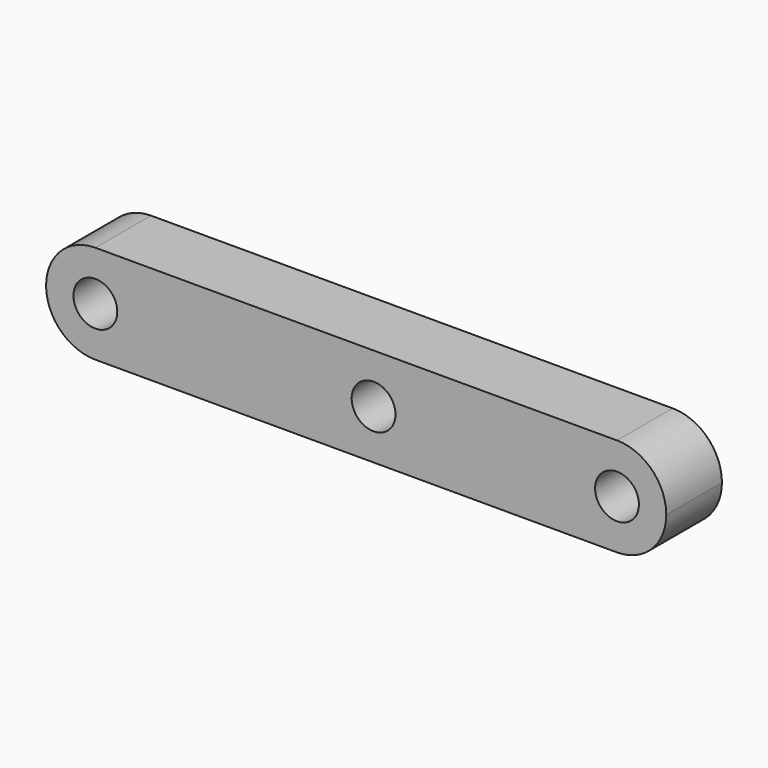
from build123d import *

# Parameters (mm, degrees)
F0_R     = 4
F1_DEPTH = 12.7


# Not quite as in the source:
# - a feature names something its author has since deleted; it is built from what else it names


with BuildPart() as f1:
    # F0 (on Front) → F1 (new body)
    with BuildSketch(Plane.XZ):
        with BuildLine():
            ThreePointArc((-50.8, -9), (-44.4360389693, -6.3639610307), (-41.8, 0))
            ThreePointArc((-41.8, 0), (-44.4360389693, 6.3639610307), (-50.8, 9))
            ThreePointArc((-50.8, 9), (-59.8, 0), (-50.8, -9))
        make_face()
        with Locations((-50.8, 0)):
            Circle(F0_R, mode=Mode.SUBTRACT)
        with BuildLine():
            ThreePointArc((9, 0), (6.3639610238, 6.3639610375), (-1.93e-08, 9))
            ThreePointArc((-1.93e-08, 9), (-9, -9.7e-09), (0, -9))
            ThreePointArc((0, -9), (6.3639610307, -6.3639610307), (9, 0))
        make_face()
        Circle(F0_R, mode=Mode.SUBTRACT)
        with BuildLine():
            ThreePointArc((-50.8, 9), (-44.4360389693, 6.3639610307), (-41.8, 0))
            ThreePointArc((-41.8, 0), (-44.4360389693, -6.3639610307), (-50.8, -9))
            Line((-50.8, -9), (0, -9))
            ThreePointArc((0, -9), (-9, -9.7e-09), (-1.93e-08, 9))
            Line((-1.93e-08, 9), (-50.8, 9))
        make_face()
        with BuildLine():
            Line((44.45, 9), (-1.93e-08, 9))
            ThreePointArc((-1.93e-08, 9), (6.3639610238, 6.3639610375), (9, 0))
            ThreePointArc((9, 0), (6.3639610307, -6.3639610307), (0, -9))
            Line((0, -9), (44.45, -9))
            ThreePointArc((44.45, -9), (35.45, 0), (44.45, 9))
        make_face()
        with BuildLine():
            ThreePointArc((53.45, 0), (50.8139610307, 6.3639610307), (44.45, 9))
            ThreePointArc((44.45, 9), (35.45, 0), (44.45, -9))
            ThreePointArc((44.45, -9), (50.8139610307, -6.3639610307), (53.45, 0))
        make_face()
        with Locations((44.45, 0)):
            Circle(F0_R, mode=Mode.SUBTRACT)
    extrude(amount=F1_DEPTH)


solid = f1.part
